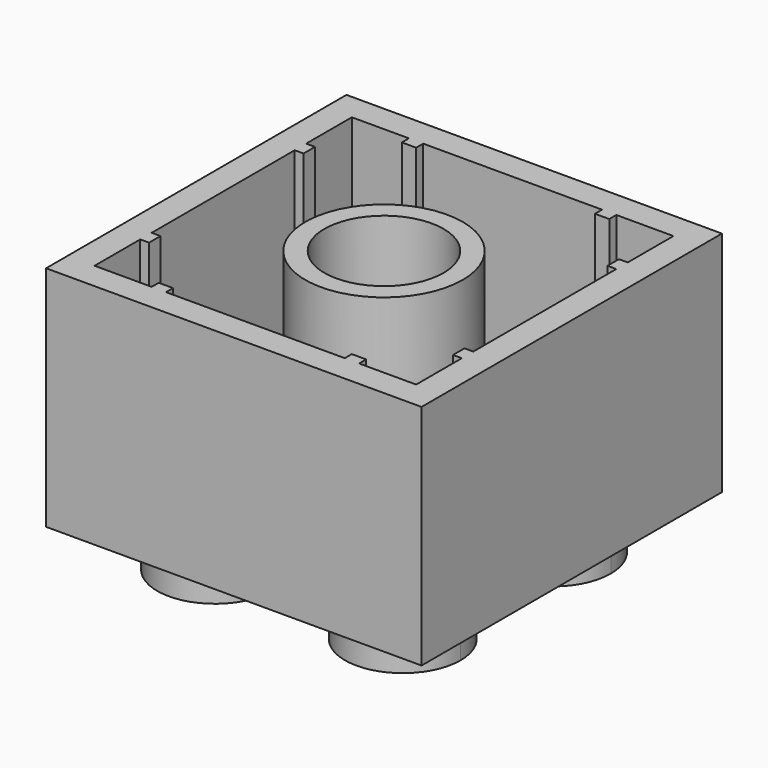
from build123d import *

# Parameters (mm, degrees)
F0_W     = 15.75
F0_H     = 15.75
F0_W_2   = 0.6
F0_H_2   = 0.37
F0_W_3   = 0.37
F0_H_3   = 0.6
F1_DEPTH = 9.55
F0_R     = 3.3
F0_R_2   = 2.5
F2_DEPTH = 1.55
F4_DEPTH = 1.9


with BuildPart() as f1:
    # F0 (on Top) → F1 (new body)
    with BuildSketch(Plane.XY):
        with Locations((7.875, 7.875)):
            Rectangle(F0_W, F0_H)
        Polygon((1.13, 12.225), (1.13, 14.62), (3.525, 14.62), (4.125, 14.62), (11.625, 14.62), (12.225, 14.62), (14.62, 14.62), (14.62, 12.225), (14.62, 11.625), (14.62, 4.125), (14.62, 3.525), (14.62, 1.13), (12.225, 1.13), (11.625, 1.13), (4.125, 1.13), (3.525, 1.13), (1.13, 1.13), (1.13, 3.525), (1.13, 4.125), (1.13, 11.625), align=None, mode=Mode.SUBTRACT)
        with Locations((3.825, 14.435)):
            Rectangle(F0_W_2, F0_H_2)
        with Locations((1.315, 11.925)):
            Rectangle(F0_W_3, F0_H_3)
        with Locations((1.315, 3.825)):
            Rectangle(F0_W_3, F0_H_3)
        with Locations((3.825, 1.315)):
            Rectangle(F0_W_2, F0_H_2)
        with Locations((11.925, 1.315)):
            Rectangle(F0_W_2, F0_H_2)
        with Locations((14.435, 3.825)):
            Rectangle(F0_W_3, F0_H_3)
        with Locations((14.435, 11.925)):
            Rectangle(F0_W_3, F0_H_3)
        with Locations((11.925, 14.435)):
            Rectangle(F0_W_2, F0_H_2)
    extrude(amount=F1_DEPTH)



with BuildPart() as f1b:
    # F0 (on Top) → F1, piece 2 (new body)
    with BuildSketch(Plane.XY):
        with Locations((7.875, 7.875)):
            Circle(F0_R)
        with Locations((7.875, 7.875)):
            Circle(F0_R_2, mode=Mode.SUBTRACT)
    extrude(amount=F1_DEPTH)


with BuildPart() as f1_1:
    add(f1.part)

    add(f1b.part)  # F2 merges F1b
    # F0 (on Top) → F2 (join)
    with BuildSketch(Plane.XY):
        Polygon((3.525, 14.62), (1.13, 14.62), (1.13, 12.225), (1.5, 12.225), (1.5, 11.625), (1.13, 11.625), (1.13, 4.125), (1.5, 4.125), (1.5, 3.525), (1.13, 3.525), (1.13, 1.13), (3.525, 1.13), (3.525, 1.5), (4.125, 1.5), (4.125, 1.13), (11.625, 1.13), (11.625, 1.5), (12.225, 1.5), (12.225, 1.13), (14.62, 1.13), (14.62, 3.525), (14.25, 3.525), (14.25, 4.125), (14.62, 4.125), (14.62, 11.625), (14.25, 11.625), (14.25, 12.225), (14.62, 12.225), (14.62, 14.62), (12.225, 14.62), (12.225, 14.25), (11.625, 14.25), (11.625, 14.62), (4.125, 14.62), (4.125, 14.25), (3.525, 14.25), align=None)
        with Locations((7.875, 7.875)):
            Circle(F0_R, mode=Mode.SUBTRACT)
        with Locations((7.875, 7.875)):
            Circle(F0_R_2)
    extrude(amount=F2_DEPTH)

    # F3 (on face) → F4 (join)
    with BuildSketch(Plane.XY):
        with BuildLine():
            ThreePointArc((5.1239527498, 6.0524361391), (1.8449210985, 2.7120455778), (6.3625, 3.9375))
            ThreePointArc((6.3625, 3.9375), (6.2837038634, 4.5506495995), (6.0524361391, 5.1239527498))
            ThreePointArc((6.0524361391, 5.1239527498), (5.5415476221, 5.5415476221), (5.1239527498, 6.0524361391))
        make_face()
        with BuildLine():
            ThreePointArc((10.6260472502, 6.0524361391), (10.2084523779, 5.5415476221), (9.6975638609, 5.1239527498))
            ThreePointArc((9.6975638609, 5.1239527498), (11.1993504005, 1.5912961366), (14.2375, 3.9375))
            ThreePointArc((14.2375, 3.9375), (13.0379544222, 6.0300789015), (10.6260472502, 6.0524361391))
        make_face()
        with BuildLine():
            ThreePointArc((6.3625, 11.8125), (1.8449210985, 13.0379544222), (5.1239527498, 9.6975638609))
            ThreePointArc((5.1239527498, 9.6975638609), (5.5415476221, 10.2084523779), (6.0524361391, 10.6260472502))
            ThreePointArc((6.0524361391, 10.6260472502), (6.2837038634, 11.1993504005), (6.3625, 11.8125))
        make_face()
        with BuildLine():
            ThreePointArc((14.2375, 11.8125), (11.1993504005, 14.1587038634), (9.6975638609, 10.6260472502))
            ThreePointArc((9.6975638609, 10.6260472502), (10.2084523779, 10.2084523779), (10.6260472502, 9.6975638609))
            ThreePointArc((10.6260472502, 9.6975638609), (13.0379544222, 9.7199210985), (14.2375, 11.8125))
        make_face()
    extrude(amount=-F4_DEPTH)


solid = f1_1.part
